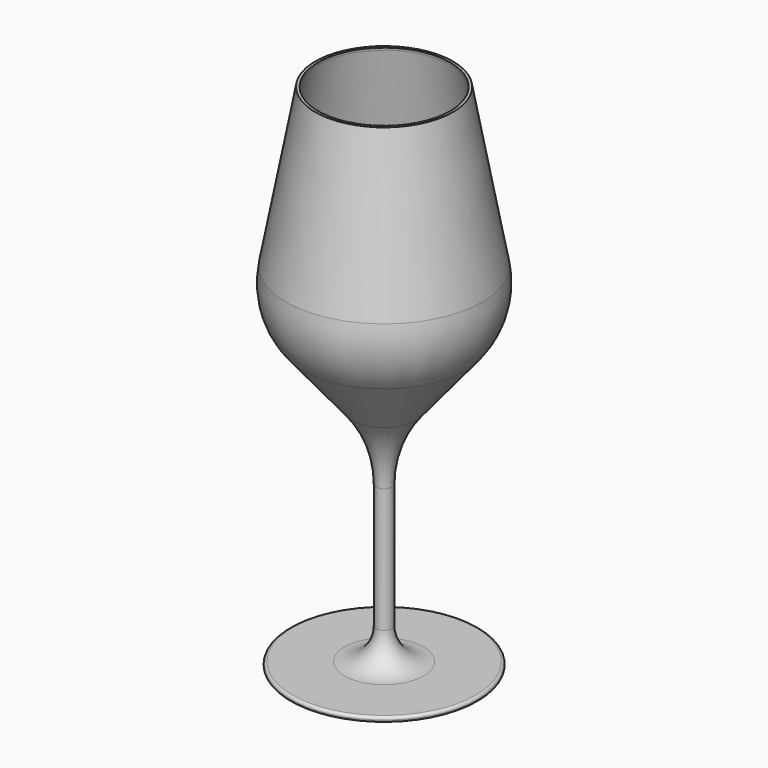
from build123d import *

# Parameters (mm, degrees)
F2_R = 1
F3_R = 0.99999


# Not quite as in the source:
# - a fillet or chamfer is up to 0.001 mm smaller than in the source, because OpenCascade refuses the exact size


with BuildPart() as f1:
    # F0 (on Front) → F1 (revolve)
    with BuildSketch(Plane.XZ):
        with BuildLine():
            Line((0, 0), (35, 0))
            Line((35, 0), (35, 2))
            Line((35, 2), (14.6711988598, 2))
            ThreePointArc((14.6711988598, 2), (6.4184150015, 5.4184150015), (3, 13.6711988598))
            Line((3, 13.6711988598), (3, 60))
            ThreePointArc((3, 60), (5.2663701885, 73.0449457567), (11.7998654023, 84.5610424876))
            Line((11.7998654023, 84.5610424876), (30.1194867973, 106.8448902178))
            ThreePointArc((30.1194867973, 106.8448902178), (35.9954931852, 118.4070626292), (36.4419899072, 131.3690039428))
            Line((36.4419899072, 131.3690039428), (25.5640022925, 190))
            Line((25.5640022925, 190), (24.5469366539, 190))
            Line((24.5469366539, 190), (24.716161279, 189.0879003841))
            Line((24.716161279, 189.0879003841), (35.4587691965, 131.186584004))
            ThreePointArc((35.4587691965, 131.186584004), (35.0271556985, 118.6567074008), (29.3470161902, 107.4799407364))
            Line((29.3470161902, 107.4799407364), (11.0273947953, 85.1960930063))
            ThreePointArc((11.0273947953, 85.1960930063), (4.3249694749, 73.3822359826), (2, 60))
            Line((2, 60), (0, 60))
            Line((0, 60), (0, 0))
        make_face()
    revolve(axis=Axis((0, 0, -18.4489581734), (0, 0, -1)))

    # F2
    f2_edges = [f1.edges().sort_by_distance(p)[0] for p in [
        (-35, 0, 2),
    ]]
    fillet(f2_edges, radius=F2_R)

    # F3 (radius 1 in the source; OpenCascade refuses exactly that, so slightly less here)
    f3_edges = [f1.edges().sort_by_distance(p)[0] for p in [
        (-35, 0, 0),
    ]]
    fillet(f3_edges, radius=F3_R)


solid = f1.part
